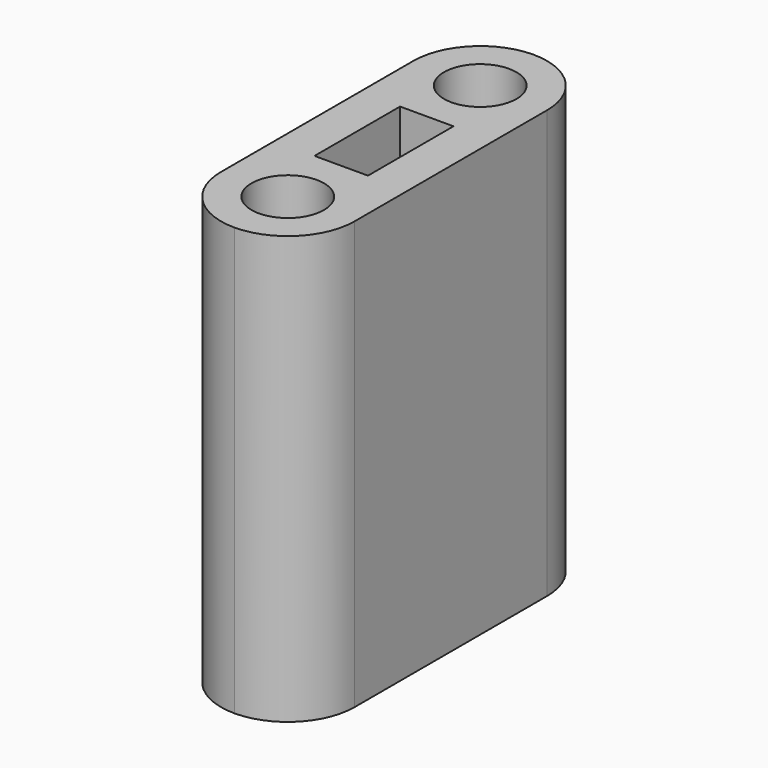
from build123d import *

# Parameters (mm, degrees)
F0_W     = 7.9375
F0_H     = 22.225
F0_W_2   = 3.175
F0_H_2   = 6.35
F1_DEPTH = 25.4
F2_R     = 2.15265
F3_DEPTH = 25.4
F4_R     = 3.96874


# Not quite as in the source:
# - a fillet or chamfer is up to 0.001 mm smaller than in the source, because OpenCascade refuses the exact size


with BuildPart() as f1:
    # F0 (on Top) → F1 (new body)
    with BuildSketch(Plane.XY):
        Rectangle(F0_W, F0_H)
        Rectangle(F0_W_2, F0_H_2, mode=Mode.SUBTRACT)
    extrude(amount=F1_DEPTH)

    # F2 (on face) → F3 (cut, through all)
    with BuildSketch(Plane.XY.offset(25.4)):
        with Locations((0, 7.14375)):
            Circle(F2_R)
        with Locations((0, -7.14375)):
            Circle(F2_R)
    extrude(amount=-F3_DEPTH, mode=Mode.SUBTRACT)

    # F4 (radius 3.96875 in the source; OpenCascade refuses exactly that, so slightly less here)
    f4_edges = [f1.edges().sort_by_distance(p)[0] for p in [
        (-3.96875, -11.1125, 12.7),
        (3.96875, -11.1125, 12.7),
        (3.96875, 11.1125, 12.7),
        (-3.96875, 11.1125, 12.7),
    ]]
    fillet(f4_edges, radius=F4_R)


solid = f1.part
